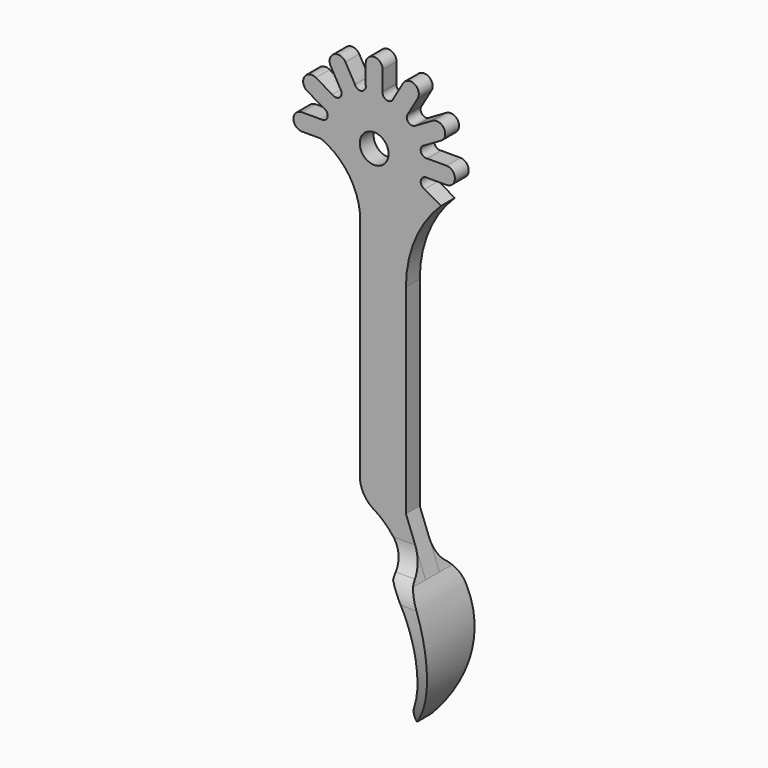
from build123d import *

# Parameters (mm, degrees)
F0_R          = 2.5
F1_DEPTH      = 1.5
F2_W          = 22
F2_H          = 33
F3_DEPTH      = 12.5
F5_DEPTH      = 25
F7_DEPTH      = 12.5
F8_W          = 13.0673529652
F8_H          = 36.5055128932
F9_DEPTH      = 12.5
F11_DEPTH     = 12.5
F12_T4_DEPTH  = 27.2917840191
F12_S6_R      = 12.1146219402
F12_T7_DEPTH  = 15
F12_T11_DEPTH = 27.2917840191
F12_S13_R     = 12.1146219402
F12_T14_DEPTH = 15
F13_T1_DEPTH  = 18.7577559022
F13_T3_DEPTH  = 22.1075441156
F13_T5_DEPTH  = 16.9663595472


# Not quite as in the source:
# - a fillet or chamfer that OpenCascade refuses, or shapes differently, is made with other operations: its cross-section is extruded or revolved along the edge and cut away or added


with BuildPart() as f1:
    # F0 (on Front) → F1 (new body, symmetric)
    with BuildSketch(Plane.XZ):
        with BuildLine():
            Line((-9.235, 1.475), (-12.525, 1.475))
            ThreePointArc((-12.525, 1.475), (-14, 0), (-12.525, -1.475))
            Line((-12.525, -1.475), (-9.235, -1.475))
            ThreePointArc((-9.235, -1.475), (-4.6343435349, -5.0926995328), (-2.4826597351, -10.5354972184))
            Line((-2.4826597351, -10.5354972184), (-2.4826597351, -54))
            Line((-2.4826597351, -54), (5.5173402649, -54))
            Line((5.5173402649, -54), (5.5173402649, -19.35))
            ThreePointArc((5.5173402649, -19.35), (7.0995621366, -11.5534976549), (11.5958851466, -4.9905749631))
            Line((11.5958851466, -4.9905749631), (8.7466615682, -3.3455749631))
            ThreePointArc((8.7466615682, -3.3455749631), (8.1072894895, -2.172712489), (9.2478806189, -1.4774032674))
            Line((9.2478806189, -1.4774032674), (12.5378806189, -1.4774032674))
            ThreePointArc((12.5378806189, -1.4774032674), (14.0128806189, -0.0024032674), (12.5378806189, 1.4725967326))
            Line((12.5378806189, 1.4725967326), (9.2478806189, 1.4725967326))
            ThreePointArc((9.2478806189, 1.4725967326), (8.1077369193, 2.168639391), (8.7478632019, 3.3410904052))
            Line((8.7478632019, 3.3410904052), (11.5970867803, 4.9860904052))
            ThreePointArc((11.5970867803, 4.9860904052), (12.1369742509, 7.0009778757), (10.1220867803, 7.5408653463))
            Line((10.1220867803, 7.5408653463), (7.2728632019, 5.8958653463))
            ThreePointArc((7.2728632019, 5.8958653463), (5.9374484648, 5.9285841208), (5.9055885801, 7.264019625))
            Line((5.9055885801, 7.264019625), (7.5505885801, 10.1132432035))
            ThreePointArc((7.5505885801, 10.1132432035), (7.0107011095, 12.1281306741), (4.9958136389, 11.5882432035))
            Line((4.9958136389, 11.5882432035), (3.3508136389, 8.739019625))
            ThreePointArc((3.3508136389, 8.739019625), (2.1779511648, 8.0996475464), (1.4826419432, 9.2402386758))
            Line((1.4826419432, 9.2402386758), (1.4826419432, 12.5302386758))
            ThreePointArc((1.4826419432, 12.5302386758), (0.0076419432, 14.0052386758), (-1.4673580568, 12.5302386758))
            Line((-1.4673580568, 12.5302386758), (-1.4673580568, 9.2402386758))
            ThreePointArc((-1.4673580568, 9.2402386758), (-2.1634007153, 8.1000949761), (-3.3358517294, 8.7402212587))
            Line((-3.3358517294, 8.7402212587), (-4.9808517294, 11.5894448372))
            ThreePointArc((-4.9808517294, 11.5894448372), (-6.9957392, 12.1293323077), (-7.5356266705, 10.1144448372))
            Line((-7.5356266705, 10.1144448372), (-5.8906266705, 7.2652212587))
            ThreePointArc((-5.8906266705, 7.2652212587), (-5.923345445, 5.9298065216), (-7.2587809492, 5.8979466369))
            Line((-7.2587809492, 5.8979466369), (-10.1080045277, 7.5429466369))
            ThreePointArc((-10.1080045277, 7.5429466369), (-12.1228919983, 7.0030591663), (-11.5830045277, 4.9881716958))
            Line((-11.5830045277, 4.9881716958), (-8.7337809492, 3.3431716958))
            ThreePointArc((-8.7337809492, 3.3431716958), (-8.0944088706, 2.1703092216), (-9.235, 1.475))
        make_face()
        Circle(F0_R, mode=Mode.SUBTRACT)
    extrude(amount=F1_DEPTH, both=True)

    # F2 (on Front) → F3 (join, symmetric)
    with BuildSketch(Plane.XZ):
        with Locations((1.5173402649, -70.5)):
            Rectangle(F2_W, F2_H)
    extrude(amount=F3_DEPTH, both=True)

    # F4 (on face) → F5 (cut)
    with BuildSketch(Plane.YZ.offset(12.5173402649)):
        with BuildLine():
            Line((-1.5, -63), (-1.5, -54))
            Line((-1.5, -54), (-12.5, -54))
            Line((-12.5, -54), (-12.5, -87))
            Line((-12.5, -87), (-0.5366366822, -87))
            ThreePointArc((-0.5366366822, -87), (-4.8712454414, -75.3910886533), (-5, -63))
            Line((-5, -63), (-1.5, -63))
        make_face()
        with BuildLine():
            Line((12.5, -54), (1.5, -54))
            Line((1.5, -54), (1.5, -63))
            Line((1.5, -63), (5, -63))
            ThreePointArc((5, -63), (4.8712454414, -75.3910886533), (0.5366366822, -87))
            Line((0.5366366822, -87), (12.5, -87))
            Line((12.5, -87), (12.5, -54))
        make_face()
    extrude(amount=-F5_DEPTH, mode=Mode.SUBTRACT)

    # F6 (on Front) → F7 (cut, symmetric)
    with BuildSketch(Plane.XZ):
        Polygon((18.106688745, -40.9277961552), (5.5173402649, -54), (8.9304046705, -63), (19.7496718225, -63), align=None)
    extrude(amount=F7_DEPTH, both=True, mode=Mode.SUBTRACT)

    # F8 (on Front) → F9 (cut, symmetric)
    with BuildSketch(Plane.XZ):
        with Locations((-9.0163362177, -72.2527564466)):
            Rectangle(F8_W, F8_H)
    extrude(amount=F9_DEPTH, both=True, mode=Mode.SUBTRACT)

    # F10 (on Front) → F11 (cut, symmetric)
    with BuildSketch(Plane.XZ):
        with BuildLine():
            ThreePointArc((8.9304046705, -63), (11.9537965274, -74.3072822088), (7.4747879279, -85.1208852732))
            Line((7.4747879279, -85.1208852732), (5.836241855, -85.1208852732))
            ThreePointArc((5.836241855, -85.1208852732), (10.1863855255, -73.9890275915), (5.4871006869, -63))
            ThreePointArc((5.4871006869, -63), (2.6973124719, -57.4417114567), (-2.4826597351, -54))
            Line((-2.4826597351, -54), (-4.7306204217, -54))
            Line((-4.7306204217, -54), (-25.9052291512, -62.5973790884))
            Line((-25.9052291512, -62.5973790884), (-15.0617258623, -81.789419055))
            Line((-15.0617258623, -81.789419055), (-7.8701885954, -94.5178027674))
            Line((-7.8701885954, -94.5178027674), (22.746598348, -94.5178027674))
            Line((22.746598348, -94.5178027674), (21.3071964681, -60.6781728566))
            Line((21.3071964681, -60.6781728566), (12.9586569965, -58.5670471191))
            Line((12.9586569965, -58.5670471191), (8.9304046705, -63))
        make_face()
    extrude(amount=F11_DEPTH, both=True, mode=Mode.SUBTRACT)

    # F12: fillet of radius 5 on 2 edges, made by hand


with BuildPart() as f12_tool2:
    # F12_s3 → F12_t4 (new body)
    with BuildSketch(Plane.YZ.offset(20.8546446882)):
        with BuildLine():
            ThreePointArc((-1.5, -58.2303039929), (-2.4688711259, -61.1883438845), (-5, -63))
            Line((-5, -63), (-1.5, -63))
            Line((-1.5, -63), (-1.5, -58.2303039929))
        make_face()
    extrude(amount=-F12_T4_DEPTH)

    split(bisect_by=Plane(origin=(-13.0799536605, 0, -4.9603026962), x_dir=(0, 1, 0), z_dir=(-0.935022628, 0, -0.35458805)), keep=Keep.TOP)

    # F12_s6 → F12_t7 (cut, symmetric)
    with BuildSketch(Plane.XZ.offset(3.2)):
        with Locations((-6.3723846527, -65.4731906992)):
            Circle(F12_S6_R)
    extrude(amount=F12_T7_DEPTH, both=True, mode=Mode.SUBTRACT)


with BuildPart() as f1_1:
    add(f1.part)

    # F12_t1: union F12_tool2
    add(f12_tool2.part)


with BuildPart() as f12_tool9:
    # F12_s10 → F12_t11 (new body)
    with BuildSketch(Plane.YZ.offset(20.8546446882)):
        with BuildLine():
            ThreePointArc((1.5, -58.2303039929), (2.4688711259, -61.1883438845), (5, -63))
            Line((5, -63), (1.5, -63))
            Line((1.5, -63), (1.5, -58.2303039929))
        make_face()
    extrude(amount=-F12_T11_DEPTH)

    split(bisect_by=Plane(origin=(-13.0799536605, 0, -4.9603026962), x_dir=(0, 1, 0), z_dir=(-0.935022628, 0, -0.35458805)), keep=Keep.TOP)

    # F12_s13 → F12_t14 (cut, symmetric)
    with BuildSketch(Plane.XZ.offset(-3.2)):
        with Locations((-6.3723846527, -65.4731906992)):
            Circle(F12_S13_R)
    extrude(amount=F12_T14_DEPTH, both=True, mode=Mode.SUBTRACT)


with BuildPart() as f1_2:
    add(f1_1.part)

    # F12_t8: union F12_tool9
    add(f12_tool9.part)

    # F13: fillet of radius 5 on 4 edges, made by hand

    # F13_s2 → F13_t1 (cut)
    with BuildSketch(Plane.XZ.offset(-9.3788779511)):
        with BuildLine():
            ThreePointArc((-0.0797737551, -55.1210357136), (-1.8407309885, -53.2994108654), (-2.4826597351, -50.8484488196))
            Line((-2.4826597351, -50.8484488196), (-2.4826597351, -54))
            ThreePointArc((-2.4826597351, -54), (-1.2504542616, -54.4945799572), (-0.0797737551, -55.1210357136))
        make_face()
    extrude(amount=F13_T1_DEPTH, mode=Mode.SUBTRACT)

    # F13_s4 → F13_t3 (cut)
    with BuildSketch(Plane.XZ.offset(-11.0537720578)):
        with BuildLine():
            ThreePointArc((7.4747879279, -85.1208852732), (7.5468124072, -83.5490676499), (8.1037496064, -82.0774633816))
            ThreePointArc((8.1037496064, -82.0774633816), (7.0618102413, -83.6675809177), (5.836241855, -85.1208852732))
            Line((5.836241855, -85.1208852732), (7.4747879279, -85.1208852732))
        make_face()
    extrude(amount=F13_T3_DEPTH, mode=Mode.SUBTRACT)

    # F13_s6 → F13_t5 (cut)
    with BuildSketch(Plane.YZ.offset(-1.2744270949)):
        with BuildLine():
            ThreePointArc((-3.4287598457, -62.1758690873), (-4.7489171353, -63.7306961181), (-5.3382927781, -65.6833708777))
            ThreePointArc((-5.3382927781, -65.6833708777), (-5.1944289727, -64.3384980615), (-5, -63))
            ThreePointArc((-5, -63), (-4.1775321149, -62.6581864352), (-3.4287598457, -62.1758690873))
        make_face()
        with BuildLine():
            ThreePointArc((5.3382927781, -65.6833708777), (4.7489171353, -63.7306961181), (3.4287598457, -62.1758690873))
            ThreePointArc((3.4287598457, -62.1758690873), (4.1775321149, -62.6581864352), (5, -63))
            ThreePointArc((5, -63), (5.1944289727, -64.3384980615), (5.3382927781, -65.6833708777))
        make_face()
    extrude(amount=F13_T5_DEPTH, mode=Mode.SUBTRACT)


solid = f1_2.part
